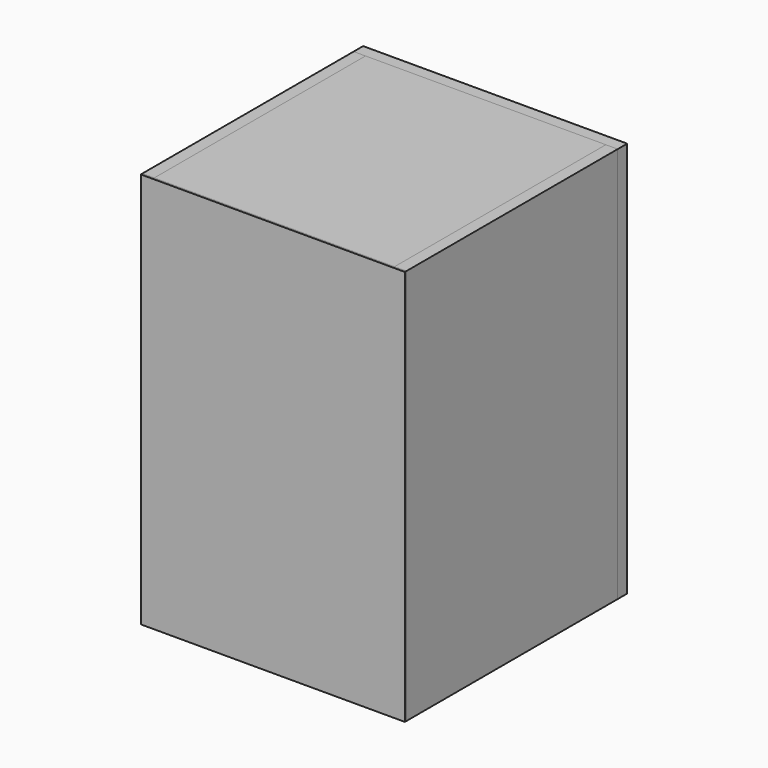
from build123d import *

# Parameters (mm, degrees)
F0_W      = 200
F0_H      = 300
F1_DEPTH  = 1.5
F2_W      = 9
F2_H      = 300
F3_DEPTH  = 200
F5_DEPTH  = 12
F7_DEPTH  = 182
F8_W      = 44.2128404975
F8_H      = 17.2260019455
F9_DEPTH  = 5
F10_W     = 200
F10_H     = 9
F11_DEPTH = 182
F12_W     = 200
F12_H     = 9
F13_DEPTH = 182
F14_W     = 200
F14_H     = 300
F15_DEPTH = 9
F16_W     = 200
F16_H     = 300
F17_DEPTH = 9
F18_R     = 40.4447812264
F19_DEPTH = 9
F20_W     = 23
F20_H     = 23
F21_DEPTH = 10
F22_W     = 23
F22_H     = 23
F23_DEPTH = 10
F24_W     = 23
F24_H     = 23
F25_DEPTH = 10


# Not quite as in the source:
# - a feature names something its author has since deleted; it is built from what else it names


with BuildPart() as f1:
    # F0 (on Front) → F1 (new body)
    with BuildSketch(Plane.XZ):
        with Locations((100, 150)):
            Rectangle(F0_W, F0_H)
    extrude(amount=F1_DEPTH)


with BuildPart() as f3:
    # F2 (on face) → F3 (new body)
    with BuildSketch(Plane(origin=(0, 0, 0), x_dir=(-1, 0, 0), z_dir=(0, 1, 0))):
        with Locations((-4.5, 150)):
            Rectangle(F2_W, F2_H)
    extrude(amount=F3_DEPTH)


with BuildPart() as f5:
    # F4 (on face) → F5 (new body)
    with BuildSketch(Plane.YZ.offset(9)):
        Polygon((24.0061823279, 108.0940887332), (0, 138.7036293745), (0, 88.1515070796), align=None)
    extrude(amount=F5_DEPTH)


with BuildPart() as f7:
    # F6 (on face) → F7 (new body)
    with BuildSketch(Plane.YZ.offset(9)):
        Polygon((0, 138.7036293745), (24.0061823279, 108.0940887332), (30.3622312434, 113.0789550838), (6.3560489155, 143.6884957251), align=None)
    extrude(amount=F7_DEPTH)


with BuildPart() as f9:
    # F8 (on face) → F9 (new body)
    with BuildSketch(Plane(origin=(0, 73.7094769341, 57.8082227142), x_dir=(-1, 0, 0), z_dir=(0, 0.7868696517, 0.6171192358))):
        with Locations((-93.7001220882, 78.8542820377)):
            Rectangle(F8_W, F8_H)
    extrude(amount=F9_DEPTH)


with BuildPart() as f11:
    # F10 (on face) → F11 (new body)
    with BuildSketch(Plane.YZ.offset(9)):
        with Locations((100, 295.5)):
            Rectangle(F10_W, F10_H)
    extrude(amount=F11_DEPTH)


with BuildPart() as f13:
    # F12 (on face) → F13 (new body)
    with BuildSketch(Plane.YZ.offset(9)):
        with Locations((100, 4.5)):
            Rectangle(F12_W, F12_H)
    extrude(amount=F13_DEPTH)


with BuildPart() as f15:
    # F14 (on face) → F15 (new body)
    with BuildSketch(Plane.YZ.offset(191)):
        with Locations((100, 150)):
            Rectangle(F14_W, F14_H)
    extrude(amount=F15_DEPTH)


with BuildPart() as f17:
    # F16 (on face) → F17 (new body)
    with BuildSketch(Plane(origin=(0, 200, 0), x_dir=(-1, 0, 0), z_dir=(0, 1, 0))):
        with Locations((-100, 150)):
            Rectangle(F16_W, F16_H)
    extrude(amount=F17_DEPTH)

    # F18 (on face) → F19 (cut)
    with BuildSketch(Plane(origin=(0, 209, 0), x_dir=(-1, 0, 0), z_dir=(0, 1, 0))):
        with Locations((-126.9655525684, 52.9041551054)):
            Circle(F18_R)
    extrude(amount=-F19_DEPTH, mode=Mode.SUBTRACT)


with BuildPart() as f21:
    # F20 (on face) → F21 (new body)
    with BuildSketch(Plane(origin=(0, 0, 0), x_dir=(1, 0, 0), z_dir=(0, 0, -1))):
        with Locations((188.5, -11.5)):
            Rectangle(F20_W, F20_H)
    extrude(amount=F21_DEPTH)


with BuildPart() as f23:
    # F22 (on face) → F23 (new body)
    with BuildSketch(Plane(origin=(0, 0, 0), x_dir=(1, 0, 0), z_dir=(0, 0, -1))):
        with Locations((11.5, -197.5752720833)):
            Rectangle(F22_W, F22_H)
    extrude(amount=F23_DEPTH)


with BuildPart() as f25:
    # F24 (on face) → F25 (new body)
    with BuildSketch(Plane(origin=(0, 0, 0), x_dir=(1, 0, 0), z_dir=(0, 0, -1))):
        with Locations((188.5, -197.5)):
            Rectangle(F24_W, F24_H)
    extrude(amount=F25_DEPTH)


solid = Compound([f1.part, f3.part, f5.part, f7.part, f9.part, f11.part, f13.part, f15.part, f17.part])
